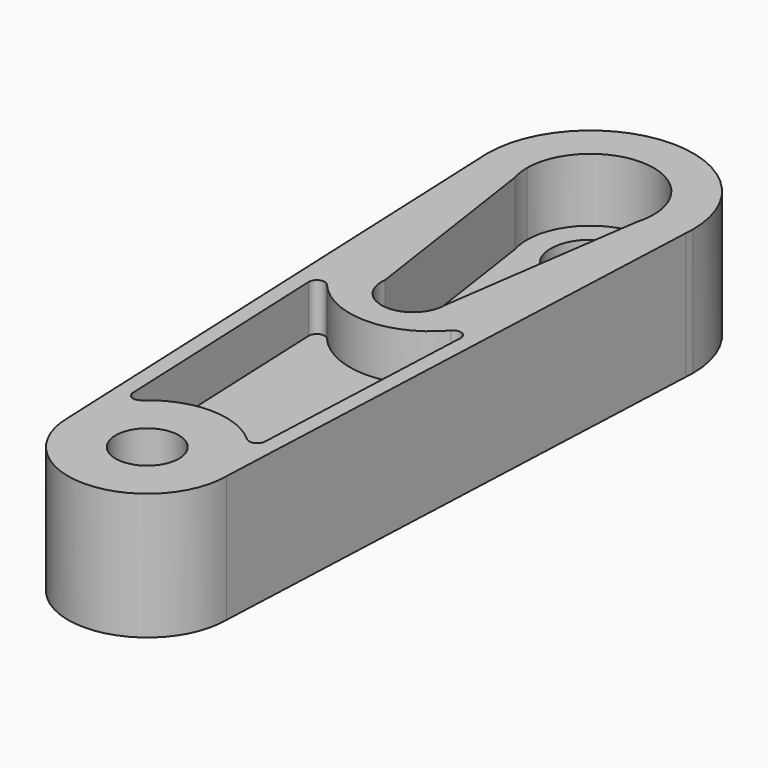
from build123d import *

# Parameters (mm, degrees)
F1_DEPTH = 8
F2_R     = 2.5
F2_R_2   = 2
F3_DEPTH = 25
F5_DEPTH = 4
F7_DEPTH = 3
F8_R     = 0.5
F9_R     = 0.5


# Not quite as in the source:
# - a feature names something its author has since deleted; it is built from what else it names


with BuildPart() as f1:
    # F0 (on Top) → F1 (new body)
    with BuildSketch(Plane.XY):
        with BuildLine():
            Line((6.4761662253, 49.1160303571), (6.5, 49.6721517667))
            ThreePointArc((6.5, 49.6721517667), (0, 56.1721517667), (-6.5, 49.6721517667))
            Line((-6.5, 49.6721517667), (-6.4761662253, 49.1160303571))
            ThreePointArc((-6.4761662253, 49.1160303571), (0, 43.1721517667), (6.4761662253, 49.1160303571))
        make_face()
        with BuildLine():
            ThreePointArc((6.4761662253, 49.1160303571), (6.4940388228, 49.3938358172), (6.5, 49.6721517667))
            Line((6.5, 49.6721517667), (6.4761662253, 49.1160303571))
        make_face()
        with BuildLine():
            Line((-6.4761662253, 49.1160303571), (-6.5, 49.6721517667))
            ThreePointArc((-6.5, 49.6721517667), (-6.4940388228, 49.3938358172), (-6.4761662253, 49.1160303571))
        make_face()
        with BuildLine():
            Line((5, 14.6721517667), (6.4761662253, 49.1160303571))
            ThreePointArc((6.4761662253, 49.1160303571), (0, 43.1721517667), (-6.4761662253, 49.1160303571))
            Line((-6.4761662253, 49.1160303571), (-5, 14.6721517667))
            ThreePointArc((-5, 14.6721517667), (0, 19.6721517667), (5, 14.6721517667))
        make_face()
        with BuildLine():
            ThreePointArc((-5, 14.6721517667), (0, 9.6721517667), (5, 14.6721517667))
            ThreePointArc((5, 14.6721517667), (0, 19.6721517667), (-5, 14.6721517667))
        make_face()
    extrude(amount=F1_DEPTH)

    # F2 (on face) → F3 (cut)
    with BuildSketch(Plane.XY.offset(8)):
        with Locations((0, 49.6721517667)):
            Circle(F2_R)
        with Locations((0, 14.6721517667)):
            Circle(F2_R_2)
    extrude(amount=-F3_DEPTH, mode=Mode.SUBTRACT)

    # F4 (on face) → F5 (cut)
    with BuildSketch(Plane.XY.offset(8)):
        with BuildLine():
            Line((3.84, 48.5521517667), (4, 49.6721517667))
            ThreePointArc((4, 49.6721517667), (0, 53.6721517667), (-4, 49.6721517667))
            Line((-4, 49.6721517667), (-3.8313540205, 48.522923169))
            ThreePointArc((-3.8313540205, 48.522923169), (0.0152402747, 45.6721808001), (3.84, 48.5521517667))
        make_face()
        with BuildLine():
            ThreePointArc((3.84, 48.5521517667), (3.9597979746, 49.1064663418), (4, 49.6721517667))
            Line((4, 49.6721517667), (3.84, 48.5521517667))
        make_face()
        with BuildLine():
            Line((-3.8313540205, 48.522923169), (-4, 49.6721517667))
            ThreePointArc((-4, 49.6721517667), (-3.9576139328, 49.0913833455), (-3.8313540205, 48.522923169))
        make_face()
        with BuildLine():
            Line((2, 35.6721517667), (3.84, 48.5521517667))
            ThreePointArc((3.84, 48.5521517667), (0.0152402747, 45.6721808001), (-3.8313540205, 48.522923169))
            Line((-3.8313540205, 48.522923169), (-1.9833417846, 35.929747119))
            ThreePointArc((-1.9833417846, 35.929747119), (0.1290667091, 37.6679828679), (2, 35.6721517667))
        make_face()
        with BuildLine():
            ThreePointArc((-1.9833417846, 35.929747119), (-0.1290667091, 33.6763206655), (2, 35.6721517667))
            ThreePointArc((2, 35.6721517667), (0.1290667091, 37.6679828679), (-1.9833417846, 35.929747119))
        make_face()
    extrude(amount=-F5_DEPTH, mode=Mode.SUBTRACT)

    # F6 (on face) → F7 (cut)
    with BuildSketch(Plane.XY.offset(8)):
        with BuildLine():
            ThreePointArc((-4.1204651564, 17.5044241573), (0, 19.6721517667), (4.1204651564, 17.5044241573))
            Line((4.1204651564, 17.5044241573), (4.8918937278, 35.5044241573))
            ThreePointArc((4.8918937278, 35.5044241573), (0, 31.9420729635), (-4.8918937278, 35.5044241573))
            Line((-4.8918937278, 35.5044241573), (-4.1204651564, 17.5044241573))
        make_face()
    extrude(amount=-F7_DEPTH, mode=Mode.SUBTRACT)

    # F8
    f8_edges = [f1.edges().sort_by_distance(p)[0] for p in [
        (4.891894, 35.504424, 6.5),
    ]]
    fillet(f8_edges, radius=F8_R)

    # F9
    f9_edges = [f1.edges().sort_by_distance(p)[0] for p in [
        (-4.891894, 35.504424, 6.5),
        (4.120465, 17.504424, 6.5),
        (-4.120465, 17.504424, 6.5),
    ]]
    fillet(f9_edges, radius=F9_R)


solid = f1.part
